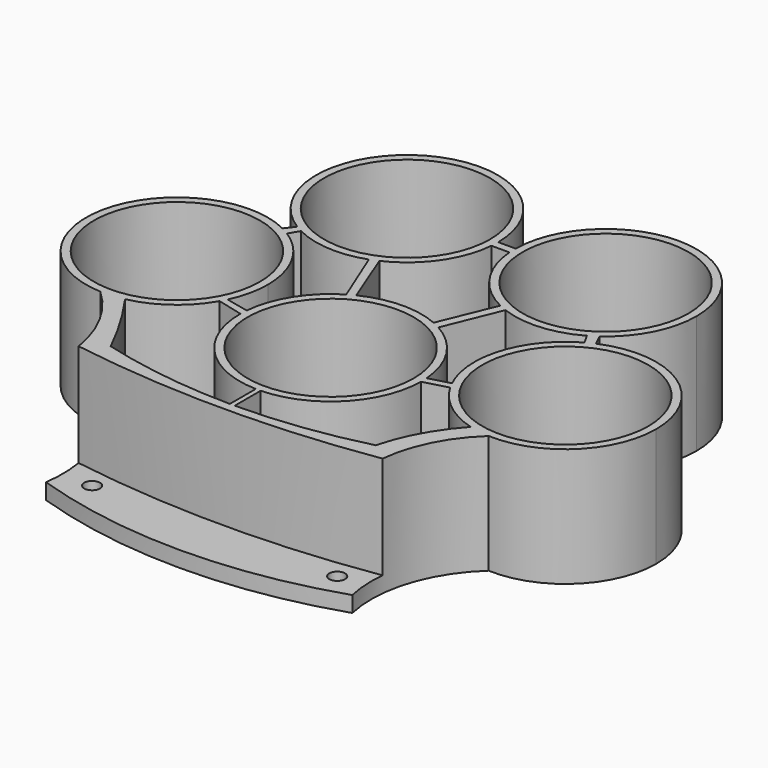
from build123d import *

# Parameters (mm, degrees)
F0_R     = 10.5
F0_R_2   = 1
F1_DEPTH = 15
F3_DEPTH = 13


# Not quite as in the source:
# - a feature names something its author has since deleted; it is built from what else it names


with BuildPart() as f1:
    # F0 (on Top) → F1 (new body)
    with BuildSketch(Plane.XY):
        with BuildLine():
            ThreePointArc((8.456539156, -32.2861623243), (7.9514162152, -32.0818291381), (7.456539156, -31.853798586))
            Line((7.456539156, -31.853798586), (4.5923320267, -38.8217959812))
            ThreePointArc((4.5923320267, -38.8217959812), (5.0983332026, -39.0569597997), (5.5923320267, -39.3163906642))
            Line((5.5923320267, -39.3163906642), (8.456539156, -32.2861623243))
        make_face()
        with BuildLine():
            ThreePointArc((5.5923320267, -39.3163906642), (5.0983332026, -39.0569597997), (4.5923320267, -38.8217959812))
            ThreePointArc((4.5923320267, -38.8217959812), (-0.2431846168, -37.8676348758), (-5.0340313362, -39.025405292))
            ThreePointArc((-5.0340313362, -39.025405292), (-5.4788213716, -39.2540536763), (-5.9132495676, -39.5018245418))
            ThreePointArc((-5.9132495676, -39.5018245418), (-9.7372709203, -43.2466031538), (-11.4521142662, -48.3166937306))
            ThreePointArc((-11.4521142662, -48.3166937306), (-11.4854214601, -48.7861903947), (-11.4994890326, -49.2566567486))
            ThreePointArc((-11.4994890326, -49.2566567486), (-8.2643935059, -57.3619252212), (-0.2699309272, -60.8618949578))
            ThreePointArc((-0.2699309272, -60.8618949578), (0.0361142384, -60.8650066318), (0.3421338242, -60.8599728394))
            ThreePointArc((0.3421338242, -60.8599728394), (8.2138697006, -57.4138113488), (11.4994866281, -49.473724691))
            ThreePointArc((11.4994866281, -49.473724691), (11.4998716563, -49.4193946208), (11.5, -49.365063338))
            ThreePointArc((11.5, -49.365063338), (11.4920706677, -48.9380835162), (11.4682936055, -48.5116925056))
            ThreePointArc((11.4682936055, -48.5116925056), (9.6904401721, -43.1726995509), (5.5923320267, -39.3163906642))
        make_face()
        with Locations((0, -49.365063338)):
            Circle(F0_R, mode=Mode.SUBTRACT)
        with BuildLine():
            Line((-5.0340313362, -39.025405292), (-7.8453759782, -31.8516950865))
            ThreePointArc((-7.8453759782, -31.8516950865), (-8.3405737258, -32.0678131455), (-8.8453759782, -32.2604332653))
            Line((-8.8453759782, -32.2604332653), (-5.9132495676, -39.5018245418))
            ThreePointArc((-5.9132495676, -39.5018245418), (-5.4788213716, -39.2540536763), (-5.0340313362, -39.025405292))
        make_face()
        with BuildLine():
            ThreePointArc((-11.4994890326, -49.2566567486), (-11.4854214601, -48.7861903947), (-11.4521142662, -48.3166937306))
            Line((-11.4521142662, -48.3166937306), (-14.3962585951, -47.6607659595))
            ThreePointArc((-14.3962585951, -47.6607659595), (-14.5881725993, -48.0436522978), (-14.7942107467, -48.4191269505))
            Line((-14.7942107467, -48.4191269505), (-11.4994890326, -49.2566567486))
        make_face()
        with BuildLine():
            Line((0.3421338242, -64.957754564), (0.3421338242, -60.8599728394))
            ThreePointArc((0.3421338242, -60.8599728394), (0.0361142384, -60.8650066318), (-0.2699309272, -60.8618949578))
            Line((-0.2699309272, -60.8618949578), (-0.2699309272, -64.9580295419))
            ThreePointArc((-0.2699309272, -64.9580295419), (0.0361017663, -64.9585994764), (0.3421338242, -64.957754564))
        make_face()
        with BuildLine():
            ThreePointArc((14.5406251326, -48.6339542886), (14.3126656094, -48.2217915649), (14.1017745949, -47.8006400066))
            Line((14.1017745949, -47.8006400066), (11.4682936055, -48.5116925056))
            ThreePointArc((11.4682936055, -48.5116925056), (11.4920706677, -48.9380835162), (11.5, -49.365063338))
            ThreePointArc((11.5, -49.365063338), (11.4998716563, -49.4193946208), (11.4994866281, -49.473724691))
            Line((11.4994866281, -49.473724691), (14.5406251326, -48.6339542886))
        make_face()
        with BuildLine():
            ThreePointArc((-18.6290237609, -32.9777593238), (-19.1442423903, -32.6707574729), (-19.6747657372, -32.391033768))
            ThreePointArc((-19.6747657372, -32.391033768), (-35.9088169714, -39.8355359758), (-25.2809881049, -54.1887337442))
            ThreePointArc((-25.2809881049, -54.1887337442), (-23.804958589, -54.1593636462), (-22.3448544462, -53.9411398473))
            ThreePointArc((-22.3448544462, -53.9411398473), (-17.9826996587, -51.9825521015), (-14.7942107467, -48.4191269505))
            ThreePointArc((-14.7942107467, -48.4191269505), (-14.5881725993, -48.0436522978), (-14.3962585951, -47.6607659595))
            ThreePointArc((-14.3962585951, -47.6607659595), (-13.5560532822, -45.2433801805), (-13.2712837616, -42.7000348848))
            ThreePointArc((-13.2712837616, -42.7000348848), (-14.6993924296, -37.1496290442), (-18.6290237609, -32.9777593238))
        make_face()
        with Locations((-24.7712837616, -42.7000348848)):
            Circle(F0_R, mode=Mode.SUBTRACT)
        with BuildLine():
            ThreePointArc((19.1164688634, -69.8349915238), (19.4845895022, -61.444857772), (23.9814303791, -54.3520248186))
            ThreePointArc((23.9814303791, -54.3520248186), (22.6698061738, -54.2185580929), (21.3820772546, -53.9358468382))
            ThreePointArc((21.3820772546, -53.9358468382), (18.3981233109, -58.1037903348), (16.5083411563, -62.8687098028))
            ThreePointArc((16.5083411563, -62.8687098028), (8.4897865212, -64.4127490141), (0.3421338242, -64.957754564))
            ThreePointArc((0.3421338242, -64.957754564), (0.0361017663, -64.9585994764), (-0.2699309272, -64.9580295419))
            ThreePointArc((-0.2699309272, -64.9580295419), (-8.785207594, -64.3721937184), (-17.154313878, -62.6955302663))
            ThreePointArc((-17.154313878, -62.6955302663), (-19.5673016908, -58.2102584784), (-22.3448544462, -53.9411398473))
            ThreePointArc((-22.3448544462, -53.9411398473), (-23.804958589, -54.1593636462), (-25.2809881049, -54.1887337442))
            ThreePointArc((-25.2809881049, -54.1887337442), (-20.5000187239, -61.334576051), (-19.5788875855, -69.8828067405))
            ThreePointArc((-19.5788875855, -69.8828067405), (-0.2273681462, -72.9674740069), (19.1164688634, -69.8349915238))
        make_face()
        with Locations((-15.5739570037, -67.6103085279)):
            Circle(F0_R_2, mode=Mode.SUBTRACT)
        with Locations((15.4391750693, -67.6299035549)):
            Circle(F0_R_2, mode=Mode.SUBTRACT)
        with BuildLine():
            ThreePointArc((-1.1916347077, -21.4227077758), (-1.1916502185, -21.4038200259), (-1.1916967507, -21.384932327))
            ThreePointArc((-1.1916967507, -21.384932327), (-18.3019531043, -11.3840660604), (-18.7497462956, -31.1976391816))
            ThreePointArc((-18.7497462956, -31.1976391816), (-18.319020566, -31.4517919016), (-17.8776520238, -31.6869770823))
            ThreePointArc((-17.8776520238, -31.6869770823), (-13.4202987359, -32.8995997215), (-8.8453759782, -32.2604332653))
            ThreePointArc((-8.8453759782, -32.2604332653), (-8.3405737258, -32.0678131455), (-7.8453759782, -31.8516950865))
            ThreePointArc((-7.8453759782, -31.8516950865), (-3.2683745706, -28.0145336524), (-1.2331773275, -22.3993113114))
            ThreePointArc((-1.2331773275, -22.3993113114), (-1.2020250565, -21.9114511274), (-1.1916347077, -21.4227077758))
        make_face()
        with Locations((-12.6916347077, -21.4227077758)):
            Circle(F0_R, mode=Mode.SUBTRACT)
        with BuildLine():
            ThreePointArc((-17.8776520238, -31.6869770823), (-18.319020566, -31.4517919016), (-18.7497462956, -31.1976391816))
            Line((-18.7497462956, -31.1976391816), (-19.6747657372, -32.391033768))
            ThreePointArc((-19.6747657372, -32.391033768), (-19.1442423903, -32.6707574729), (-18.6290237609, -32.9777593238))
            Line((-18.6290237609, -32.9777593238), (-17.8776520238, -31.6869770823))
        make_face()
        with BuildLine():
            ThreePointArc((1.0484752677, -22.3993113114), (1.0211177974, -21.8924785724), (1.0161513841, -21.384932327))
            Line((1.0161513841, -21.384932327), (-1.1916967507, -21.384932327))
            ThreePointArc((-1.1916967507, -21.384932327), (-1.1916502185, -21.4038200259), (-1.1916347077, -21.4227077758))
            ThreePointArc((-1.1916347077, -21.4227077758), (-1.2020250565, -21.9114511274), (-1.2331773275, -22.3993113114))
            Line((-1.2331773275, -22.3993113114), (1.0484752677, -22.3993113114))
        make_face()
        with BuildLine():
            ThreePointArc((19.2285761762, -30.8633233175), (22.7488768974, -26.7724999097), (24.0152835635, -21.5262090793))
            ThreePointArc((24.0152835635, -21.5262090793), (12.5859232723, -10.0264260365), (1.0161513841, -21.384932327))
            ThreePointArc((1.0161513841, -21.384932327), (1.0211177974, -21.8924785724), (1.0484752677, -22.3993113114))
            ThreePointArc((1.0484752677, -22.3993113114), (2.9958137546, -27.97831684), (7.456539156, -31.853798586))
            ThreePointArc((7.456539156, -31.853798586), (7.9514162152, -32.0818291381), (8.456539156, -32.2861623243))
            ThreePointArc((8.456539156, -32.2861623243), (13.3927953164, -32.9926807739), (18.1640607336, -31.5432603661))
            ThreePointArc((18.1640607336, -31.5432603661), (18.7056608481, -31.2179183751), (19.2285761762, -30.8633233175))
        make_face()
        with Locations((12.5152835635, -21.5262090793)):
            Circle(F0_R, mode=Mode.SUBTRACT)
        with BuildLine():
            Line((19.9216749616, -32.3085805793), (19.2285761762, -30.8633233175))
            ThreePointArc((19.2285761762, -30.8633233175), (18.7056608481, -31.2179183751), (18.1640607336, -31.5432603661))
            Line((18.1640607336, -31.5432603661), (18.8762154015, -32.8253023654))
            ThreePointArc((18.8762154015, -32.8253023654), (19.3923910412, -32.5536807799), (19.9216749616, -32.3085805793))
        make_face()
        with BuildLine():
            ThreePointArc((35.9878958911, -42.8631827235), (30.8021044444, -33.251691146), (19.9216749616, -32.3085805793))
            ThreePointArc((19.9216749616, -32.3085805793), (19.3923910412, -32.5536807799), (18.8762154015, -32.8253023654))
            ThreePointArc((18.8762154015, -32.8253023654), (13.5312723299, -39.3699893221), (14.1017745949, -47.8006400066))
            ThreePointArc((14.1017745949, -47.8006400066), (14.3126656094, -48.2217915649), (14.5406251326, -48.6339542886))
            ThreePointArc((14.5406251326, -48.6339542886), (17.4435150212, -51.9531056143), (21.3820772546, -53.9358468382))
            ThreePointArc((21.3820772546, -53.9358468382), (22.6698061738, -54.2185580929), (23.9814303791, -54.3520248186))
            ThreePointArc((23.9814303791, -54.3520248186), (32.4385451291, -51.1720440591), (35.9878958911, -42.8631827235))
        make_face()
        with Locations((24.4878958911, -42.8631827235)):
            Circle(F0_R, mode=Mode.SUBTRACT)
    extrude(amount=F1_DEPTH)

    # F2 (on face) → F3 (cut)
    with BuildSketch(Plane.XY.offset(15)):
        with BuildLine():
            Line((-25.4734057233, -63.6063340564), (-25.4734057233, -67.6063340564))
            ThreePointArc((-25.4734057233, -67.6063340564), (-0.2376476142, -73.3314436205), (24.9858820328, -67.5526964371))
            Line((24.9858820328, -67.5526964371), (24.9858820328, -63.5526964371))
            ThreePointArc((24.9858820328, -63.5526964371), (-0.2410172674, -66.1614613713), (-25.4734057233, -63.6063340564))
        make_face()
    extrude(amount=-F3_DEPTH, mode=Mode.SUBTRACT)


solid = f1.part
